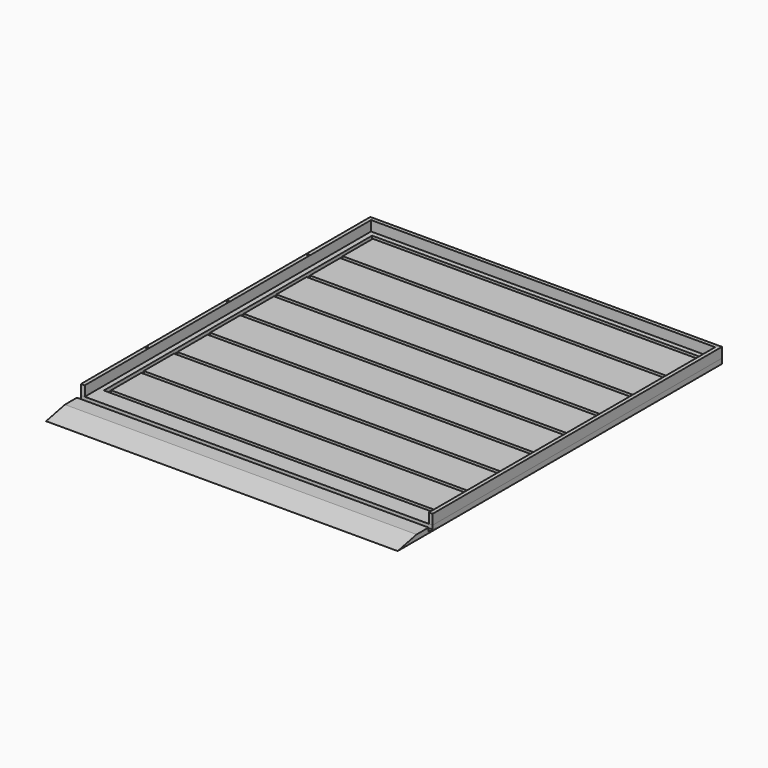
from build123d import *

# Parameters (mm, degrees)
F0_W      = 889
F0_H      = 914.4
F1_DEPTH  = 12.7
F2_W      = 12.7
F2_H      = 3.175
F3_DEPTH  = 889.001
F5_DEPTH  = 889
F7_DEPTH  = 25.4
F8_DEPTH  = 25.4
F6_W      = 869.95
F6_H      = 9.525
F9_DEPTH  = 25.4
F10_W     = 844.55
F10_H     = 847.725
F10_W_2   = 825.4364864731
F10_H_2   = 95.25
F10_W_3   = 825.5
F11_DEPTH = 9.525
F13_R     = 3.175
F13_R_2   = 1.905
F14_DEPTH = 6.35
F15_DEPTH = 25.4


with BuildPart() as f1:
    # F0 (on Top) → F1 (new body)
    with BuildSketch(Plane.XY):
        Rectangle(F0_W, F0_H)
    extrude(amount=F1_DEPTH)

    # F2 (on face) → F3 (cut, through all)
    with BuildSketch(Plane.YZ.offset(444.5)):
        with Locations((-450.85, 1.5875)):
            Rectangle(F2_W, F2_H)
    extrude(amount=-F3_DEPTH, mode=Mode.SUBTRACT)

    # F10 (on face) → F11 (cut)
    with BuildSketch(Plane.XY.offset(12.7)):
        with Locations((0, 11.1125)):
            Rectangle(F10_W, F10_H)
        with Locations((1.1747297096, -355.6)):
            Rectangle(F10_W_2, F10_H_2, mode=Mode.SUBTRACT)
        with Locations((0, -250.825)):
            Rectangle(F10_W_3, F10_H_2, mode=Mode.SUBTRACT)
        with Locations((1.1747297096, -146.05)):
            Rectangle(F10_W_2, F10_H_2, mode=Mode.SUBTRACT)
        with Locations((0, -41.275)):
            Rectangle(F10_W_3, F10_H_2, mode=Mode.SUBTRACT)
        with Locations((1.1747297096, 63.5)):
            Rectangle(F10_W_2, F10_H_2, mode=Mode.SUBTRACT)
        with Locations((0, 168.275)):
            Rectangle(F10_W_3, F10_H_2, mode=Mode.SUBTRACT)
        with Locations((1.1747297096, 273.05)):
            Rectangle(F10_W_2, F10_H_2, mode=Mode.SUBTRACT)
        with Locations((0, 377.825)):
            Rectangle(F10_W_3, F10_H_2, mode=Mode.SUBTRACT)
    extrude(amount=-F11_DEPTH, mode=Mode.SUBTRACT)


with BuildPart() as f5:
    # F4 (on face) → F5 (new body, through all)
    with BuildSketch(Plane.YZ.offset(444.5)):
        Polygon((-469.9, 12.7), (-508, 12.7), (-567.5374269485, 0), (-444.5, 0), (-444.5, 3.175), (-457.2, 3.175), (-469.9, 3.175), align=None)
    extrude(amount=-F5_DEPTH)


with BuildPart() as f7:
    # F6 (on face) → F7 (new body)
    with BuildSketch(Plane.XY.offset(12.7)):
        Polygon((434.975, -457.2), (444.5, -457.2), (444.5, 457.2), (434.975, 457.2), (434.975, 447.675), align=None)
    extrude(amount=F7_DEPTH)


with BuildPart() as f8:
    # F6 (on face) → F8 (new body)
    with BuildSketch(Plane.XY.offset(12.7)):
        Polygon((-444.5, -457.2), (-434.975, -457.2), (-434.975, 447.675), (-434.975, 457.2), (-444.5, 457.2), align=None)
    extrude(amount=F8_DEPTH)

    # F13 (on face) → F14 (cut)
    with BuildSketch(Plane.XY.offset(38.1)):
        with Locations((-439.7375, -254)):
            Circle(F13_R)
        with Locations((-439.7375, -254)):
            Circle(F13_R_2, mode=Mode.SUBTRACT)
        with Locations((-439.7375, 0)):
            Circle(F13_R)
        with Locations((-439.7375, 0)):
            Circle(F13_R_2, mode=Mode.SUBTRACT)
        with Locations((-439.7375, 254)):
            Circle(F13_R)
        with Locations((-439.7375, 254)):
            Circle(F13_R_2, mode=Mode.SUBTRACT)
        with Locations((439.7375, 254)):
            Circle(F13_R)
        with Locations((439.7375, 254)):
            Circle(F13_R_2, mode=Mode.SUBTRACT)
        with Locations((439.7375, 0)):
            Circle(F13_R)
        with Locations((439.7375, 0)):
            Circle(F13_R_2, mode=Mode.SUBTRACT)
        with Locations((439.7375, -254)):
            Circle(F13_R)
        with Locations((439.7375, -254)):
            Circle(F13_R_2, mode=Mode.SUBTRACT)
    extrude(amount=-F14_DEPTH, mode=Mode.SUBTRACT)

    # F15 (cut, through all): faces of the model
    f15_faces = [f8.faces().sort_by_distance(p)[0] for p in [
        (-439.7375, -254, 38.1),
        (-439.7375, 0, 38.1),
        (-439.7375, 254, 38.1),
    ]]
    extrude(f15_faces, amount=-F15_DEPTH, mode=Mode.SUBTRACT)


with BuildPart() as f9:
    # F6 (on face) → F9 (new body)
    with BuildSketch(Plane.XY.offset(12.7)):
        with Locations((0, 452.4375)):
            Rectangle(F6_W, F6_H)
    extrude(amount=F9_DEPTH)


solid = Compound([f1.part, f5.part, f7.part, f8.part, f9.part])
